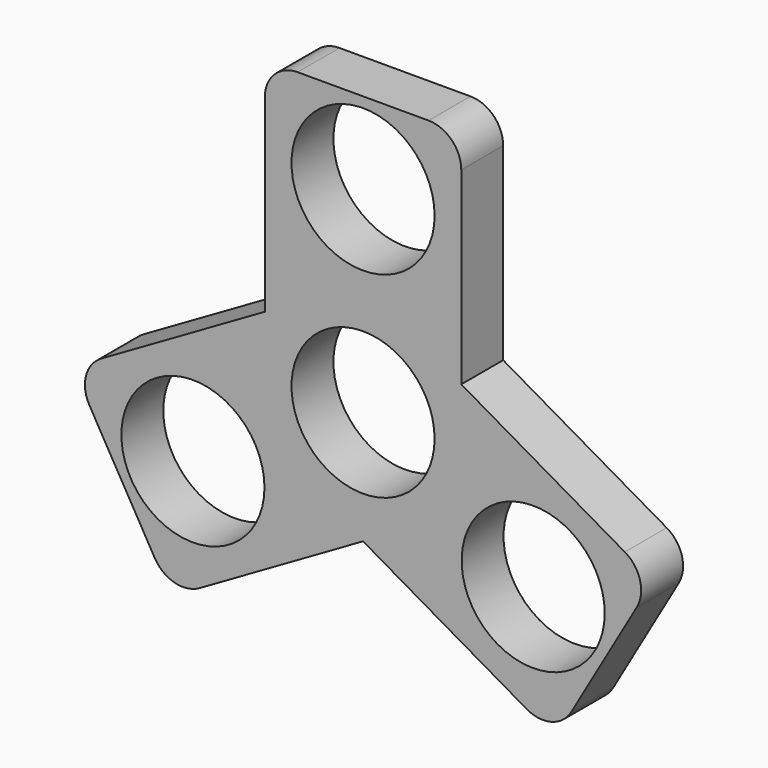
from build123d import *

# Parameters (mm, degrees)
F0_R     = 10.925
F1_DEPTH = 8


with BuildPart() as f1:
    # F0 (on Front) → F1 (new body)
    with BuildSketch(Plane.XZ):
        Polygon((1107.5254678726, 519.4568690529), (1115.874832778, 524.2773771286), (1099.1761029672, 524.2773771286), align=None)
        Polygon((1114.1761029672, 550.2581392421), (1122.5254678726, 535.7966150151), (1122.5254678726, 545.4376311664), align=None)
        Polygon((1092.5254678726, 545.4376311664), (1092.5254678726, 535.7966150151), (1100.874832778, 550.2581392421), align=None)
        with BuildLine():
            Line((1114.1761029672, 550.2581392421), (1122.5254678726, 545.4376311664))
            Line((1122.5254678726, 545.4376311664), (1122.5254678726, 574.2773771286))
            ThreePointArc((1122.5254678726, 574.2773771286), (1121.0610017786, 577.8129110345), (1117.5254678726, 579.2773771286))
            Line((1117.5254678726, 579.2773771286), (1097.5254678726, 579.2773771286))
            ThreePointArc((1097.5254678726, 579.2773771286), (1093.9899339667, 577.8129110345), (1092.5254678726, 574.2773771286))
            Line((1092.5254678726, 574.2773771286), (1092.5254678726, 545.4376311664))
            Line((1092.5254678726, 545.4376311664), (1100.874832778, 550.2581392421))
            Line((1100.874832778, 550.2581392421), (1104.2001503253, 556.0177581854))
            Line((1104.2001503253, 556.0177581854), (1107.5254678726, 554.0978852043))
            Line((1107.5254678726, 554.0978852043), (1110.8507854199, 556.0177581854))
            Line((1110.8507854199, 556.0177581854), (1114.1761029672, 550.2581392421))
        make_face()
        with Locations((1107.5254678726, 566.7773771286)):
            Circle(F0_R, mode=Mode.SUBTRACT)
        with BuildLine():
            Line((1107.5254678726, 519.4568690529), (1099.1761029672, 524.2773771286))
            Line((1099.1761029672, 524.2773771286), (1092.5254678726, 524.2773771286))
            Line((1092.5254678726, 524.2773771286), (1092.5254678726, 528.1171230908))
            Line((1092.5254678726, 528.1171230908), (1089.2001503253, 530.0369960718))
            Line((1089.2001503253, 530.0369960718), (1092.5254678726, 535.7966150151))
            Line((1092.5254678726, 535.7966150151), (1092.5254678726, 545.4376311664))
            Line((1092.5254678726, 545.4376311664), (1067.5495152307, 531.0177581854))
            ThreePointArc((1067.5495152307, 531.0177581854), (1065.2198860993, 527.981726392), (1065.7193882118, 524.1876311664))
            Line((1065.7193882118, 524.1876311664), (1075.7193882118, 506.8671230908))
            ThreePointArc((1075.7193882118, 506.8671230908), (1078.7554200052, 504.5374939593), (1082.5495152307, 505.0369960718))
            Line((1082.5495152307, 505.0369960718), (1107.5254678726, 519.4568690529))
        make_face()
        with Locations((1081.5447057591, 521.7773771286)):
            Circle(F0_R, mode=Mode.SUBTRACT)
        Polygon((1099.1761029672, 524.2773771286), (1115.874832778, 524.2773771286), (1122.5254678726, 528.1171230908), (1122.5254678726, 535.7966150151), (1114.1761029672, 550.2581392421), (1107.5254678726, 554.0978852043), (1100.874832778, 550.2581392421), (1092.5254678726, 535.7966150151), (1092.5254678726, 528.1171230908), align=None)
        with Locations((1107.5254678726, 536.7773771286)):
            Circle(F0_R, mode=Mode.SUBTRACT)
        Polygon((1100.874832778, 550.2581392421), (1107.5254678726, 554.0978852043), (1104.2001503253, 556.0177581854), align=None)
        Polygon((1107.5254678726, 554.0978852043), (1114.1761029672, 550.2581392421), (1110.8507854199, 556.0177581854), align=None)
        Polygon((1115.874832778, 524.2773771286), (1122.5254678726, 524.2773771286), (1122.5254678726, 528.1171230908), align=None)
        Polygon((1089.2001503253, 530.0369960718), (1092.5254678726, 528.1171230908), (1092.5254678726, 535.7966150151), align=None)
        Polygon((1092.5254678726, 524.2773771286), (1099.1761029672, 524.2773771286), (1092.5254678726, 528.1171230908), align=None)
        with BuildLine():
            Line((1122.5254678726, 528.1171230908), (1122.5254678726, 524.2773771286))
            Line((1122.5254678726, 524.2773771286), (1115.874832778, 524.2773771286))
            Line((1115.874832778, 524.2773771286), (1107.5254678726, 519.4568690529))
            Line((1107.5254678726, 519.4568690529), (1132.5014205145, 505.0369960718))
            ThreePointArc((1132.5014205145, 505.0369960718), (1136.29551574, 504.5374939593), (1139.3315475335, 506.8671230908))
            Line((1139.3315475335, 506.8671230908), (1149.3315475335, 524.1876311664))
            ThreePointArc((1149.3315475335, 524.1876311664), (1149.831049646, 527.981726392), (1147.5014205145, 531.0177581854))
            Line((1147.5014205145, 531.0177581854), (1122.5254678726, 545.4376311664))
            Line((1122.5254678726, 545.4376311664), (1122.5254678726, 535.7966150151))
            Line((1122.5254678726, 535.7966150151), (1125.8507854199, 530.0369960718))
            Line((1125.8507854199, 530.0369960718), (1122.5254678726, 528.1171230908))
        make_face()
        with Locations((1133.5062299862, 521.7773771286)):
            Circle(F0_R, mode=Mode.SUBTRACT)
        Polygon((1122.5254678726, 535.7966150151), (1122.5254678726, 528.1171230908), (1125.8507854199, 530.0369960718), align=None)
    extrude(amount=F1_DEPTH)


solid = f1.part
